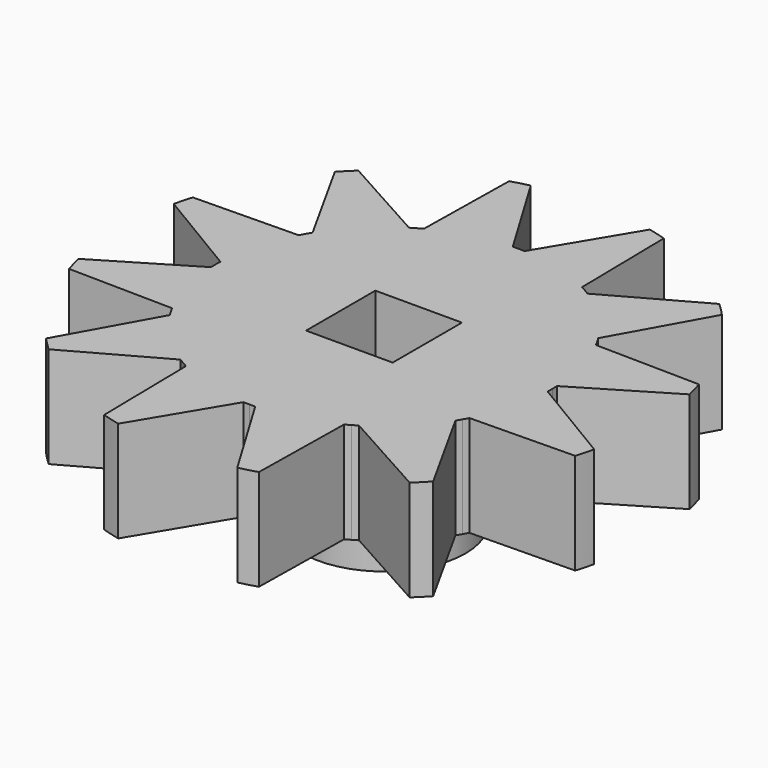
from build123d import *

# Parameters (mm, degrees)
F0_R            = 11
F1_DEPTH        = 4.2
F3_DEPTH        = 4.201
F3_COPIES_COUNT = 12
F5_R            = 3.3858769499
F6_DEPTH        = 3
F7_W            = 3.6
F7_H            = 3.6
F8_DEPTH        = 7.201


# Not quite as in the source:
# - a pattern or mirror of a feature is missing from the dataset's text; its kind, count and spacing are read off the source's solid


with BuildPart() as f1:
    # F0 (on Top) → F1 (new body)
    with BuildSketch(Plane.XY):
        Circle(F0_R)
    extrude(amount=F1_DEPTH)

    # F2 (on face) → F3 (cut, through all)
    with BuildSketch(Plane(origin=(0, 0, 0), x_dir=(1, 0, 0), z_dir=(0, 0, -1))):
        with BuildLine():
            ThreePointArc((-0.2442964769, 6.9957357891), (-0.1221668451, 6.9989338661), (0, 7))
            Line((0, 7), (0, 11))
            ThreePointArc((0, 11), (-1.2452353514, 10.9292904124), (-2.4744615978, 10.7180707126))
            Line((-2.4744615978, 10.7180707126), (-0.2442964769, 6.9957357891))
        make_face()
        with BuildLine():
            Line((0, 11), (0, 7))
            ThreePointArc((0, 7), (0.1221668451, 6.9989338661), (0.2442964769, 6.9957357891))
            Line((0.2442964769, 6.9957357891), (2.4744615978, 10.7180707126))
            ThreePointArc((2.4744615978, 10.7180707126), (1.2452353514, 10.9292904124), (0, 11))
        make_face()
    f3 = extrude(amount=-F3_DEPTH, mode=Mode.SUBTRACT)

    # F3_copies: F3 ×12 about axis
    f3_copies_axis = Axis((0, 0, 0), (0, 0, 1))
    for i in range(1, F3_COPIES_COUNT):
        add(f3.rotate(f3_copies_axis, i * 360 / F3_COPIES_COUNT), mode=Mode.SUBTRACT)

    # F5 (on face) → F6 (join)
    with BuildSketch(Plane(origin=(0, 0, 0), x_dir=(1, 0, 0), z_dir=(0, 0, -1))):
        Circle(F5_R)
    extrude(amount=F6_DEPTH)

    # F7 (on face) → F8 (cut, through all)
    with BuildSketch(Plane(origin=(0, 0, -3), x_dir=(1, 0, 0), z_dir=(0, 0, -1))):
        Rectangle(F7_W, F7_H)
    extrude(amount=-F8_DEPTH, mode=Mode.SUBTRACT)


solid = f1.part
